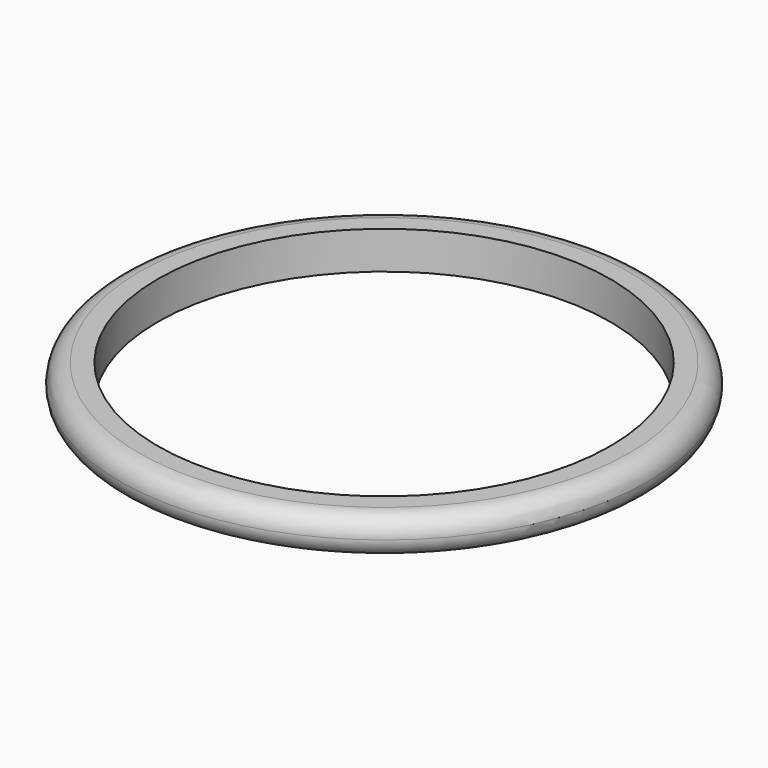
from build123d import *

# Parameters (mm, degrees)
F0_R     = 11.1125
F0_R_2   = 9.525
F1_DEPTH = 1.5875
F2_R     = 0.79374


# Not quite as in the source:
# - a fillet or chamfer is up to 0.001 mm smaller than in the source, because OpenCascade refuses the exact size


with BuildPart() as f1:
    # F0 (on Top) → F1 (new body)
    with BuildSketch(Plane.XY):
        Circle(F0_R)
        Circle(F0_R_2, mode=Mode.SUBTRACT)
    extrude(amount=F1_DEPTH)

    # F2 (radius 0.79375 in the source; OpenCascade refuses exactly that, so slightly less here)
    f2_edges = [f1.edges().sort_by_distance(p)[0] for p in [
        (-11.1125, 0, 0),
        (-11.1125, 0, 1.5875),
    ]]
    fillet(f2_edges, radius=F2_R)


solid = f1.part
